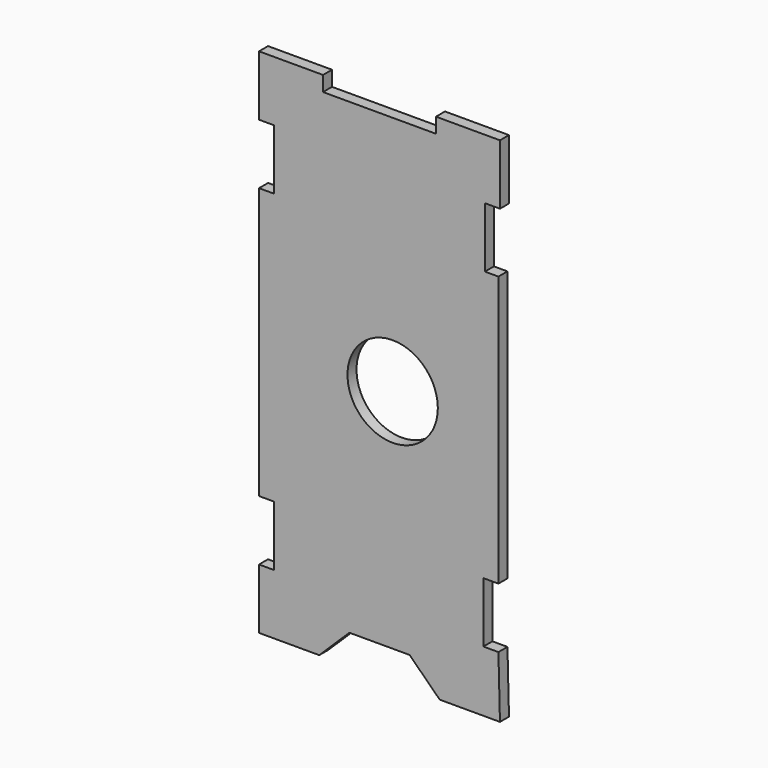
from build123d import *

# Parameters (mm, degrees)
F0_R     = 76.2
F1_DEPTH = 19.05


# Not quite as in the source:
# - a length typed as a fraction of an inch, garbled in the dataset ("3 / 203.2 mm" for 3/8 in), is restored
# - a feature names something its author has since deleted; it is built from what else it names


with BuildPart() as f1:
    # F0 (on Front) → F1 (new body)
    with BuildSketch(Plane.XZ):
        Polygon((-277.4270822048, 25.2823245883), (-277.4270822048, -76.3176754117), (-175.8270822048, -76.3176754117), (-125.0270822048, -26.4387615025), (-23.4270822048, -26.4387615025), (27.3729177952, -76.3176754117), (128.9729177952, -76.3176754117), (126.3909138083, 26.5286043286), (100.9909138083, 26.5286043286), (100.9909138083, 128.1286043286), (126.3909138083, 128.1286043286), (126.3909138083, 584.0823245883), (103.5729177952, 584.0823245883), (103.5729177952, 685.6823245883), (128.9729177952, 685.6823245883), (128.9729177952, 787.2823245883), (21.0229177952, 787.2823245883), (21.0229177952, 761.8823245883), (-169.4770822048, 761.8823245883), (-169.4770822048, 787.2823245883), (-277.4270822048, 787.2823245883), (-277.4270822048, 685.6823245883), (-252.0270822048, 685.6823245883), (-252.0270822048, 584.0823245883), (-277.4270822048, 584.0823245883), (-277.4270822048, 126.8823245883), (-252.0270822048, 126.8823245883), (-252.0270822048, 25.2823245883), align=None)
        with Locations((-52.0020822048, 355.4823245883)):
            Circle(F0_R, mode=Mode.SUBTRACT)
    extrude(amount=F1_DEPTH)


solid = f1.part
